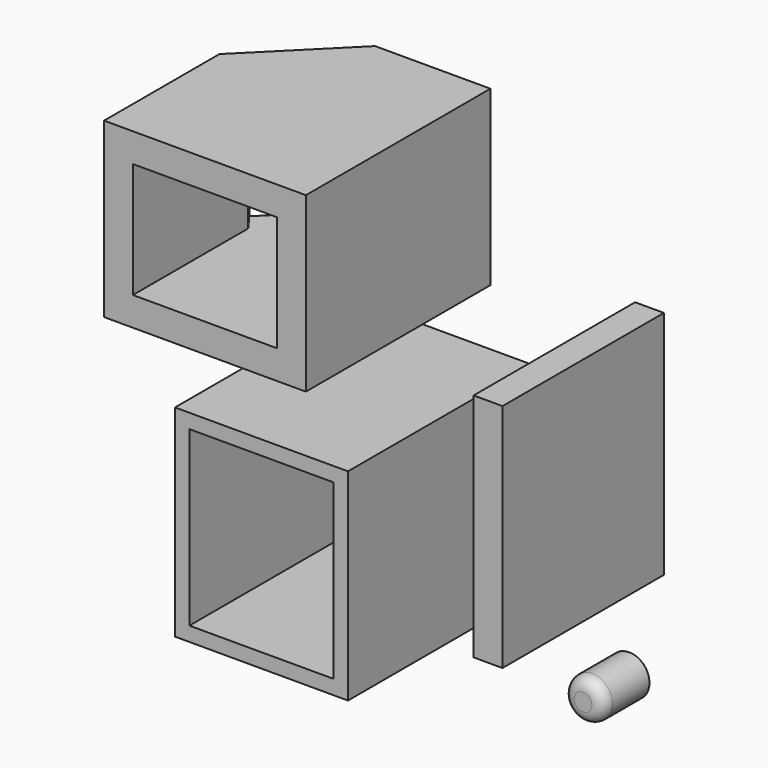
from build123d import *

# Parameters (mm, degrees)
F0_W        = 12.7
F0_H        = 101.6
F1_DEPTH    = 88.9
F0_W_2      = 88.9
F0_H_2      = 76.2
F0_W_3      = 63.5
F0_H_3      = 50.8
F2_DEPTH    = 101.6
F3_T1_DEPTH = 272.162243683
F4_T1_DEPTH = 50.8
F5_W        = 76.2
F5_H        = 88.9
F6_DEPTH    = 101.6
F7_T        = -6.35
F8_R        = 8.961281468
F9_DEPTH    = 25.4
F10_R       = 5.08


# Not quite as in the source:
# - a fillet or chamfer that OpenCascade refuses, or shapes differently, is made with other operations: its cross-section is extruded or revolved along the edge and cut away or added


with BuildPart() as f1:
    # F0 (on Front) → F1 (new body)
    with BuildSketch(Plane.XZ):
        with Locations((51.5435934067, -23.9115703218)):
            Rectangle(F0_W, F0_H)
    extrude(amount=F1_DEPTH)


with BuildPart() as f2:
    # F0 (on Front) → F2 (new body)
    with BuildSketch(Plane.XZ):
        with Locations((-62.9948227882, 50.8801213741)):
            Rectangle(F0_W_2, F0_H_2)
        with Locations((-62.9948227882, 50.8801213741)):
            Rectangle(F0_W_3, F0_H_3, mode=Mode.SUBTRACT)
    extrude(amount=F2_DEPTH)

    # F3: chamfer of 38.1 on 1 edges, made by hand

    # F3_s2 → F3_t1 (cut)
    with BuildSketch(Plane.XY.offset(-85.2010004674)):
        Polygon((-107.4448227882, -38.1), (-69.3448227882, 0), (-107.4448227882, 0), align=None)
    extrude(amount=F3_T1_DEPTH, mode=Mode.SUBTRACT)

    # F4: chamfer of 12.7 x 7.62 on 1 edges, made by hand

    # F4_s2 → F4_t1 (cut)
    with BuildSketch(Plane.XY.offset(25.4801213741)):
        Polygon((-100.1329764609, -30.7881536727), (-94.7448227882, -38.1), (-94.7448227882, -25.4), align=None)
    extrude(amount=F4_T1_DEPTH, mode=Mode.SUBTRACT)


with BuildPart() as f6:
    # F5 (on Front) → F6 (new body)
    with BuildSketch(Plane.XZ):
        with Locations((-38.1, -56.5309760347)):
            Rectangle(F5_W, F5_H)
    extrude(amount=F6_DEPTH)

    # F7
    f7_openings = [f6.faces().sort_by_distance(p)[0] for p in [
        (-38.1, -101.6, -56.530976),
    ]]
    offset(amount=F7_T, openings=f7_openings)


with BuildPart() as f9:
    # F8 (on Front) → F9 (new body)
    with BuildSketch(Plane.XZ):
        with Locations((42.5848402083, -118.6522245407)):
            Circle(F8_R)
    extrude(amount=F9_DEPTH)

    # F10
    f10_edges = [f9.edges().sort_by_distance(p)[0] for p in [
        (33.623559, -25.4, -118.652225),
    ]]
    fillet(f10_edges, radius=F10_R)


solid = Compound([f1.part, f2.part, f6.part, f9.part])
